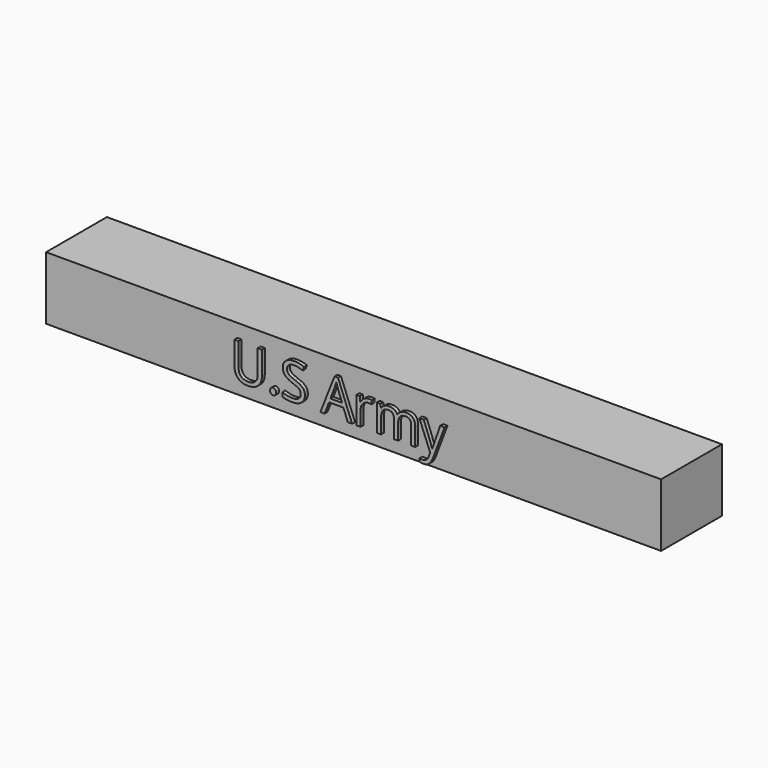
from build123d import *

# Parameters (mm, degrees)
F0_W         = 129.4672563672
F0_H         = 13.2713494822
F1_DEPTH     = 16.002
F2_R         = 1.9812
F3_DEPTH     = 124.46
F4_TEXT_SIZE = 10.5657433677
F5_DEPTH     = 0.762


# Not quite as in the source:
# - Text() gives the source's letters only with a copy of the font that has no kerning and outlines rounded to 1/6400 em; it was checked with that copy


with BuildPart() as f1:
    # F0 (on Front) → F1 (new body)
    with BuildSketch(Plane.XZ):
        with Locations((11.9346641004, 6.6356747411)):
            Rectangle(F0_W, F0_H)
    extrude(amount=F1_DEPTH)

    # F2 (on face) → F3 (cut)
    with BuildSketch(Plane(origin=(-52.7989640832, 0, 0), x_dir=(0, -1, 0), z_dir=(-1, 0, 0))):
        with Locations((7.4555040337, 6.2512867153)):
            Circle(F2_R)
    extrude(amount=-F3_DEPTH, mode=Mode.SUBTRACT)

    # F4 (on face) → F5 (join)
    with BuildSketch(Plane.XZ.offset(16.002)):
        with Locations((-13.4960161522, 2.9288195074)):
            Text('U.S Army', F4_TEXT_SIZE, font='Open Sans', text_align=(TextAlign.LEFT, TextAlign.BOTTOM))
    extrude(amount=F5_DEPTH)


solid = f1.part
